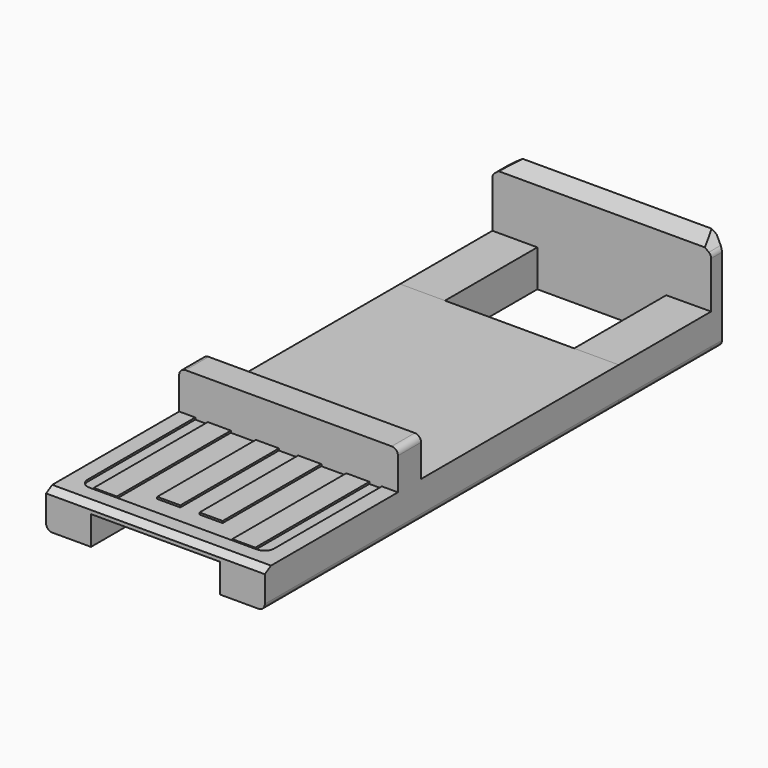
from build123d import *

# Parameters (mm, degrees)
F1_DEPTH     = 23
F2_R         = 0.325
F3_SIZE2     = 0.2309401077
F3_SIZE      = 0.4
F5_DEPTH     = 7
F7_DEPTH     = 1
F8_T1_DEPTH  = 2.6245000769
F8_T3_DEPTH  = 1.8050905296
F9_W         = 11.37
F9_H         = 1.5
F10_DEPTH    = 2
F11_R        = 0.325
F12_T1_DEPTH = 6.7216810245
F14_DEPTH    = 0.1
F15_W        = 1.2
F15_H        = 6.41
F15_H_2      = 7.41
F16_DEPTH    = 0.1
F17_T1_DEPTH = 15.6207881718


# Not quite as in the source:
# - a fillet or chamfer that OpenCascade refuses, or shapes differently, is made with other operations: its cross-section is extruded or revolved along the edge and cut away or added


with BuildPart() as f1:
    # F0 (on Front) → F1 (new body)
    with BuildSketch(Plane.XZ):
        Polygon((0, 1.92), (0, 0), (2.335, 0), (2.335, 1.5), (9.035, 1.5), (9.035, 0), (11.37, 0), (11.37, 1.92), align=None)
    extrude(amount=F1_DEPTH)

    # F2
    f2_edges = [f1.edges().sort_by_distance(p)[0] for p in [
        (11.37, -11.5, 0),
        (0, -11.5, 0),
    ]]
    fillet(f2_edges, radius=F2_R)

    # F3
    f3_edges = [f1.edges().sort_by_distance(p)[0] for p in [
        (5.685, -23, 1.92),
    ]]
    f3_side = f1.faces().sort_by_distance((5.685, -11.5, 1.92))[0]
    chamfer(f3_edges, length=F3_SIZE, length2=F3_SIZE2, reference=f3_side)

    # F4 (on Front) → F5 (join)
    with BuildSketch(Plane.XZ):
        with BuildLine():
            ThreePointArc((0, 0.325), (0.0951902961, 0.0951902961), (0.325, 0))
            Line((0.325, 0), (2.335, 0))
            Line((2.335, 0), (2.335, 1.9198597874))
            Line((2.335, 1.9198597874), (0, 1.92))
            Line((0, 1.92), (0, 0.325))
        make_face()
        with BuildLine():
            Line((9.035, 1.9067822723), (9.035, 0))
            Line((9.035, 0), (11.045, 0))
            ThreePointArc((11.045, 0), (11.2748097039, 0.0951902961), (11.37, 0.325))
            Line((11.37, 0.325), (11.37, 1.92))
            Line((11.37, 1.92), (9.035, 1.9067822723))
        make_face()
    extrude(amount=-F5_DEPTH)

    # F6 (on face) → F7 (join)
    with BuildSketch(Plane(origin=(0, 7, 0), x_dir=(-1, 0, 0), z_dir=(0, 1, 0))):
        with BuildLine():
            Line((-11.37, 0), (0, 0))
            Line((0, 0), (0, 4.5))
            ThreePointArc((0, 4.5), (-0.4145888759, 4.8120524944), (-0.8462680731, 5.1))
            Line((-0.8462680731, 5.1), (-10.5237319269, 5.1))
            ThreePointArc((-10.5237319269, 5.1), (-10.9554111241, 4.8120524944), (-11.37, 4.5))
            Line((-11.37, 4.5), (-11.37, 0))
        make_face()
    extrude(amount=-F7_DEPTH)

    # F8: fillet of radius 0.325 on 4 edges, made by hand

    # F8_s2 → F8_t1 (cut)
    with BuildSketch(Plane.XZ.offset(-7.8122500385)):
        with BuildLine():
            ThreePointArc((-0.0001, 0.3249), (0.0950902961, 0.0950902961), (0.3249, -0.0001))
            Line((0.3249, -0.0001), (0.3249, -0.0066))
            ThreePointArc((0.3249, -0.0066), (0.16245, -0.0065), (0, -0.0065))
            Line((0, -0.0065), (-0.0065, 0))
            ThreePointArc((-0.0065, 0), (-0.0065, 0.16245), (-0.0066, 0.3249))
            Line((-0.0066, 0.3249), (-0.0001, 0.3249))
        make_face()
        with BuildLine():
            ThreePointArc((11.3701, 0.3249), (11.2749097039, 0.0950902961), (11.0451, -0.0001))
            Line((11.0451, -0.0001), (11.0451, -0.0066))
            ThreePointArc((11.0451, -0.0066), (11.20755, -0.0065), (11.37, -0.0065))
            Line((11.37, -0.0065), (11.3765, 0))
            ThreePointArc((11.3765, 0), (11.3765, 0.16245), (11.3766, 0.3249))
            Line((11.3766, 0.3249), (11.3701, 0.3249))
        make_face()
    extrude(amount=F8_T1_DEPTH, mode=Mode.SUBTRACT)

    # F8_s4 → F8_t3 (cut)
    with BuildSketch(Plane.XZ.offset(-7.4025452648)):
        with BuildLine():
            ThreePointArc((-0.0001, 4.3418793672), (0.0333071199, 4.4854014639), (0.1266605677, 4.5994179613))
            Line((0.1266605677, 4.5994179613), (0.122695779, 4.6045687332))
            ThreePointArc((0.122695779, 4.6045687332), (0.0591315692, 4.5550650769), (-0.0040551807, 4.5050799123))
            Line((-0.0040551807, 4.5050799123), (-0.0065, 4.5))
            ThreePointArc((-0.0065, 4.5), (-0.0065, 4.4209396836), (-0.0066, 4.3418793672))
            Line((-0.0066, 4.3418793672), (-0.0001, 4.3418793672))
        make_face()
        with BuildLine():
            ThreePointArc((11.2433394323, 4.5994179613), (11.3366928801, 4.4854014639), (11.3701, 4.3418793672))
            Line((11.3701, 4.3418793672), (11.3766, 4.3418793672))
            ThreePointArc((11.3766, 4.3418793672), (11.3765, 4.4209396836), (11.3765, 4.5))
            Line((11.3765, 4.5), (11.3740551807, 4.5050799123))
            ThreePointArc((11.3740551807, 4.5050799123), (11.3108684308, 4.5550650769), (11.247304221, 4.6045687332))
            Line((11.247304221, 4.6045687332), (11.2433394323, 4.5994179613))
        make_face()
    extrude(amount=F8_T3_DEPTH, mode=Mode.SUBTRACT)

    # F9 (on face) → F10 (join)
    with BuildSketch(Plane.XY.offset(1.92)):
        with Locations((5.685, -13.6)):
            Rectangle(F9_W, F9_H)
    extrude(amount=F10_DEPTH)

    # F11
    f11_edges = [f1.edges().sort_by_distance(p)[0] for p in [
        (0, -13.6, 3.92),
        (11.37, -13.6, 3.92),
    ]]
    fillet(f11_edges, radius=F11_R)

    # F12: chamfer of 0.3 x 0.5196152423 on 2 edges, made by hand

    # F12_s2 → F12_t1 (cut)
    with BuildSketch(Plane.XY.offset(-1.0274508288)):
        Polygon((10.8503847577, 7), (11.37, 6.7), (11.37, 7), align=None)
        Polygon((0, 6.7), (0.5196152423, 7), (0, 7), align=None)
    extrude(amount=F12_T1_DEPTH, mode=Mode.SUBTRACT)

    # F13 (on face) → F14 (cut)
    with BuildSketch(Plane.XY.offset(1.92)):
        with BuildLine():
            Line((10.535, -14.35), (0.835, -14.35))
            Line((0.835, -14.35), (0.835, -21.35))
            ThreePointArc((0.835, -21.35), (0.9814466094, -21.7035533906), (1.335, -21.85))
            Line((1.335, -21.85), (10.035, -21.85))
            ThreePointArc((10.035, -21.85), (10.3885533906, -21.7035533906), (10.535, -21.35))
            Line((10.535, -21.35), (10.535, -14.35))
        make_face()
    extrude(amount=-F14_DEPTH, mode=Mode.SUBTRACT)

    # F15 (on face) → F16 (join, through all)
    with BuildSketch(Plane.XY.offset(1.82)):
        with Locations((4.585, -17.555)):
            Rectangle(F15_W, F15_H)
        with Locations((2.085, -18.055)):
            Rectangle(F15_W, F15_H_2)
        with Locations((9.285, -18.055)):
            Rectangle(F15_W, F15_H_2)
        with Locations((6.785, -17.555)):
            Rectangle(F15_W, F15_H)
    extrude(amount=F16_DEPTH)

    # F17: chamfer of 0.35 x 1.1447984165 on 1 edges, made by hand

    # F17_s2 → F17_t1 (cut)
    with BuildSketch(Plane.YZ.offset(-2.1253940859)):
        Polygon((6, 4.75), (7.1447984165, 5.1), (6, 5.1), align=None)
    extrude(amount=F17_T1_DEPTH, mode=Mode.SUBTRACT)


solid = f1.part
